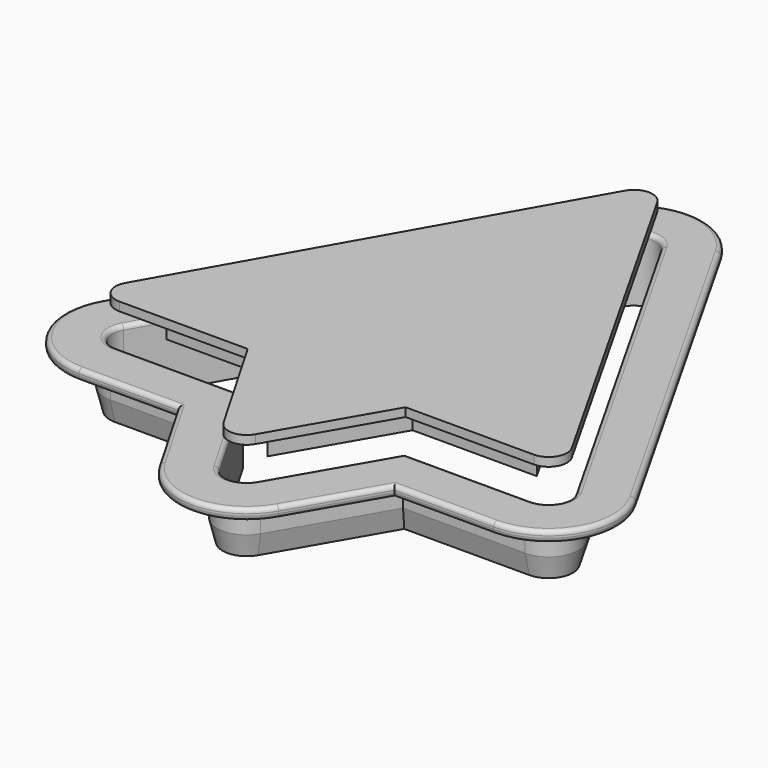
from build123d import *

# Parameters (mm, degrees)
F1_DEPTH     = 2.5
F2_DEPTH     = 15
F0_R         = 2.1252371371
F3_DEPTH     = 15
F4_DEPTH     = 7
F5_T1_DEPTH  = 97.369641179
F5_T3_DEPTH  = 97.369641179
F5_T6_ANGLE  = 119.5382480003
F5_T10_DEPTH = 41.2120527161
F5_T15_DEPTH = 40.6442974674
F5_T18_ANGLE = 120.9235039995
F5_T20_ANGLE = 119.5382480003
F5_T24_DEPTH = 41.2120527161
F5_T29_DEPTH = 40.6442974674
F5_T32_ANGLE = 119.912621019
F5_T37_DEPTH = 40.6442974674
F5_T42_DEPTH = 41.2120527161
F5_T50_DEPTH = 41.2120527161
F5_T55_DEPTH = 40.6442974674
F6_R         = 1
F8_DEPTH     = 25
F9_DEPTH     = 6


# Not quite as in the source:
# - a fillet or chamfer that OpenCascade refuses, or shapes differently, is made with other operations: its cross-section is extruded or revolved along the edge and cut away or added


with BuildPart() as f1:
    # F0 (on Top) → F1 (new body)
    with BuildSketch(Plane.XY):
        with BuildLine():
            Line((65.2872159777, -47.6204884105), (17.2835486697, 37.0937072612))
            ThreePointArc((17.2835486697, 37.0937072612), (3.4454325214, 45.1576695615), (-10.3926836269, 37.0937072612))
            Line((-10.3926836269, 37.0937072612), (-58.3963509349, -47.6204884105))
            ThreePointArc((-58.3963509349, -47.6204884105), (-58.3005499368, -63.4700527455), (-44.5582347866, -71.3673080758))
            Line((-44.5582347866, -71.3673080758), (-21.5553492686, -71.3673080758))
            Line((-21.5553492686, -71.3673080758), (-10.3229719901, -90.7881414994))
            ThreePointArc((-10.3229719901, -90.7881414994), (3.4454325214, -98.7303359177), (17.2138370329, -90.7881414994))
            Line((17.2138370329, -90.7881414994), (28.4462143115, -71.3673080758))
            Line((28.4462143115, -71.3673080758), (51.4490998294, -71.3673080758))
            ThreePointArc((51.4490998294, -71.3673080758), (65.1914149796, -63.4700527455), (65.2872159777, -47.6204884105))
        make_face()
        with BuildLine():
            ThreePointArc((-2.5142515817, 32.629359488), (3.4454325214, 36.1022793142), (9.4051166245, 32.629359488))
            Line((9.4051166245, 32.629359488), (57.4087839325, -52.0848361837))
            ThreePointArc((57.4087839325, -52.0848361837), (57.36752516, -58.9107939655), (51.4490998294, -62.3119178285))
            Line((51.4490998294, -62.3119178285), (23.2226846121, -62.3119178285))
            Line((23.2226846121, -62.3119178285), (9.3750937999, -86.254467817))
            ThreePointArc((9.3750937999, -86.254467817), (3.4454325214, -89.6749456705), (-2.4842287571, -86.254467817))
            Line((-2.4842287571, -86.254467817), (-16.3318195693, -62.3119178285))
            Line((-16.3318195693, -62.3119178285), (-44.5582347866, -62.3119178285))
            ThreePointArc((-44.5582347866, -62.3119178285), (-50.4766601172, -58.9107939655), (-50.5179188897, -52.0848361837))
            Line((-50.5179188897, -52.0848361837), (-2.5142515817, 32.629359488))
        make_face(mode=Mode.SUBTRACT)
    extrude(amount=-F1_DEPTH)

    # F0 (on Top) → F2 (join)
    with BuildSketch(Plane.XY):
        with BuildLine():
            Line((57.4087839325, -52.0848361837), (9.4051166245, 32.629359488))
            ThreePointArc((9.4051166245, 32.629359488), (3.4454325214, 36.1022793142), (-2.5142515817, 32.629359488))
            Line((-2.5142515817, 32.629359488), (-50.5179188897, -52.0848361837))
            ThreePointArc((-50.5179188897, -52.0848361837), (-50.4766601172, -58.9107939655), (-44.5582347866, -62.3119178285))
            Line((-44.5582347866, -62.3119178285), (-16.3318195693, -62.3119178285))
            Line((-16.3318195693, -62.3119178285), (-2.4842287571, -86.254467817))
            ThreePointArc((-2.4842287571, -86.254467817), (3.4454325214, -89.6749456705), (9.3750937999, -86.254467817))
            Line((9.3750937999, -86.254467817), (23.2226846121, -62.3119178285))
            Line((23.2226846121, -62.3119178285), (51.4490998294, -62.3119178285))
            ThreePointArc((51.4490998294, -62.3119178285), (57.36752516, -58.9107939655), (57.4087839325, -52.0848361837))
        make_face()
        with BuildLine():
            ThreePointArc((-0.9047013933, 31.7173008756), (3.4454325214, 34.2522785787), (7.7955664361, 31.7173008756))
            Line((7.7955664361, 31.7173008756), (55.7992337441, -52.9968947961))
            ThreePointArc((55.7992337441, -52.9968947961), (55.769117855, -57.9793451968), (51.4490998294, -60.461917093))
            Line((51.4490998294, -60.461917093), (22.155526431, -60.461917093))
            Line((22.155526431, -60.461917093), (7.773651968, -85.3282460399))
            ThreePointArc((7.773651968, -85.3282460399), (3.4454325214, -87.8249449349), (-0.8827869252, -85.3282460399))
            Line((-0.8827869252, -85.3282460399), (-15.2646613882, -60.461917093))
            Line((-15.2646613882, -60.461917093), (-44.5582347866, -60.461917093))
            ThreePointArc((-44.5582347866, -60.461917093), (-48.8782528122, -57.9793451968), (-48.9083687013, -52.9968947961))
            Line((-48.9083687013, -52.9968947961), (-0.9047013933, 31.7173008756))
        make_face(mode=Mode.SUBTRACT)
    extrude(amount=-F2_DEPTH)

    # F5: chamfer of 5 x 1.25 on 10 edges, made by hand

    # F5_s2 → F5_t1 (cut)
    with BuildSketch(Plane(origin=(13.3845186224, 23.6202522252, 0), x_dir=(0, 0, 1), z_dir=(-0.4930044594, -0.8700267829, 0))):
        Polygon((-10, 18.273885949), (-15, 17.023885949), (-15, 18.273885949), align=None)
    extrude(amount=F5_T1_DEPTH, mode=Mode.SUBTRACT)

    # F5_s4 → F5_t3 (cut)
    with BuildSketch(Plane(origin=(36.2939968422, -64.0496220939, 0), x_dir=(0, 0, 1), z_dir=(-0.4930044594, 0.8700267829, 0))):
        Polygon((-10, 24.2691230939), (-15, 23.0191230939), (-15, 24.2691230939), align=None)
    extrude(amount=F5_T3_DEPTH, mode=Mode.SUBTRACT)

    # F5_s5 → F5_t6 (revolve, cut)
    with BuildSketch(Plane(origin=(-34.6191486856, -61.0939434465, 0), x_dir=(0, 0, 1), z_dir=(0.4930044594, 0.8700267829, 0))):
        Polygon((-10, -18.273885949), (-15, -17.023885949), (-15, -18.273885949), align=None)
    revolve(axis=Axis((-44.5582347866, -55.461917093, -15), (0, 0, 1)), revolution_arc=F5_T6_ANGLE, mode=Mode.SUBTRACT)


with BuildPart() as f3:
    # F0 (on Top) → F3 (new body)
    with BuildSketch(Plane.XY):
        with BuildLine():
            Line((55.7992337441, -52.9968947961), (7.7955664361, 31.7173008756))
            ThreePointArc((7.7955664361, 31.7173008756), (3.4454325214, 34.2522785787), (-0.9047013933, 31.7173008756))
            Line((-0.9047013933, 31.7173008756), (-48.9083687013, -52.9968947961))
            ThreePointArc((-48.9083687013, -52.9968947961), (-48.8782528122, -57.9793451968), (-44.5582347866, -60.461917093))
            Line((-44.5582347866, -60.461917093), (-15.2646613882, -60.461917093))
            Line((-15.2646613882, -60.461917093), (-0.8827869252, -85.3282460399))
            ThreePointArc((-0.8827869252, -85.3282460399), (3.4454325214, -87.8249449349), (7.773651968, -85.3282460399))
            Line((7.773651968, -85.3282460399), (22.155526431, -60.461917093))
            Line((22.155526431, -60.461917093), (51.4490998294, -60.461917093))
            ThreePointArc((51.4490998294, -60.461917093), (55.769117855, -57.9793451968), (55.7992337441, -52.9968947961))
        make_face()
        Polygon((-39.4101028585, -52.4619175743), (3.4454325214, 23.1671418995), (46.3009679013, -52.4619175743), (17.5407904627, -52.4619175743), (3.4454325214, -76.8328581005), (-10.6499254199, -52.4619175743), align=None, mode=Mode.SUBTRACT)
        Polygon((46.3009679013, -52.4619175743), (3.4454325214, 23.1671418995), (-39.4101028585, -52.4619175743), (-10.6499254199, -52.4619175743), (3.4454325214, -76.8328581005), (17.5407904627, -52.4619175743), align=None)
        Polygon((-35.3587796887, -50.1010675165), (3.4454325214, 18.3784427043), (42.2496447315, -50.1010675165), (16.1789529211, -50.1010675165), (3.4454325214, -72.1173844943), (-9.2880878783, -50.1010675165), align=None, mode=Mode.SUBTRACT)
        Polygon((42.2496447315, -50.1010675165), (3.4454325214, 18.3784427043), (-35.3587796887, -50.1010675165), (-9.2880878783, -50.1010675165), (3.4454325214, -72.1173844943), (16.1789529211, -50.1010675165), align=None)
        with Locations((-14.878096059, -27.4075604975)):
            Circle(F0_R, mode=Mode.SUBTRACT)
        Polygon((-12.8765748814, -42.689666152), (-12.8765748814, -35.4246795177), (-11.767576843, -35.4246795177), (-9.1813210194, -41.2681277739), (-6.5903947689, -35.4246795177), (-5.4648038931, -35.4246795177), (-5.4648038931, -42.689666152), (-6.3942293637, -42.689666152), (-6.3942293637, -36.9316674769), (-8.9472681284, -42.689666152), (-9.4033638015, -42.689666152), (-11.9518004358, -36.9316674769), (-11.9518004358, -42.689666152), align=None, mode=Mode.SUBTRACT)
        Polygon((-2.7839182876, -42.689666152), (-3.7133437581, -42.689666152), (-3.7133437581, -35.4246795177), (-2.5877528824, -35.4246795177), (0.0031733681, -41.2681277739), (2.5894291918, -35.4246795177), (3.6984272301, -35.4246795177), (3.6984272301, -42.689666152), (2.7736527845, -42.689666152), (2.7736527845, -36.9316674769), (0.2252161503, -42.689666152), (-0.2308795229, -42.689666152), (-2.7839182876, -36.9316674769), align=None, mode=Mode.SUBTRACT)
        Polygon((7.0893075317, -39.0533059835), (4.8316721804, -35.4246795177), (5.9392736293, -35.4246795177), (7.673623506, -38.402441889), (9.4814058393, -35.4246795177), (10.5444919318, -35.4246795177), (8.2598868757, -39.0533059835), (10.5607574806, -42.689666152), (9.4446605071, -42.689666152), (7.6309749857, -39.6361723542), (5.8071413077, -42.689666152), (4.6372665092, -42.689666152), align=None, mode=Mode.SUBTRACT)
        Polygon((10.8218248934, -36.2534187734), (10.8218248934, -35.4246795177), (13.1533117965, -35.4246795177), (13.1533117965, -36.2534187734), (12.4322017655, -36.2534187734), (12.4322017655, -41.8955646455), (13.1625505164, -41.8955646455), (13.1625505164, -42.689666152), (10.8218248934, -42.689666152), (10.8218248934, -41.8955646455), (11.5015460178, -41.8955646455), (11.5015460178, -36.2534187734), align=None, mode=Mode.SUBTRACT)
        Polygon((16.0190779716, -42.689666152), (13.3707774803, -35.4246795177), (14.4054275006, -35.4246795177), (16.5070295334, -41.5401048958), (18.6662711203, -35.4246795177), (19.673185423, -35.4246795177), (16.9846378267, -42.689666152), align=None, mode=Mode.SUBTRACT)
        with Locations((21.7689611018, -27.4075604975)):
            Circle(F0_R, mode=Mode.SUBTRACT)
        with BuildLine():
            Line((-7.565066684, -27.4075604975), (-7.565066684, -11.1319441348))
            Line((-7.565066684, -11.1319441348), (-2.4298110511, -11.1319441348))
            add(Edge.make_bspline(
                [(-2.4298110511, -11.1319441348), (-2.3662628859, -11.1277319227), (-2.1761521622, -11.1151306665), (-1.2327957206, -11.2783416604), (-0.5211634317, -11.547496959), (0.2299466047, -11.9524717121), (0.7848702041, -12.4353144963), (1.2318193278, -13.0031014274), (1.5460073362, -13.6587083311), (1.6843174255, -14.3229828977), (1.7077365425, -15.0653349157), (1.646054142, -15.8432341211), (1.1886971111, -17.0127703282), (0.6250596434, -17.7036813267), (-0.2627651619, -18.4198849126), (-0.854730177, -18.6291207008), (-1.1375576723, -18.729088828)],
                knots=[0, 0, 0, 0, 0.0388828811, 0.1163220472, 0.1889199067, 0.2620977169, 0.3309604833, 0.3989173697, 0.4669571129, 0.5329803689, 0.6011841527, 0.6727074701, 0.7614150711, 0.8383080917, 0.9227472633, 1, 1, 1, 1], degree=3))
            add(Edge.make_bspline(
                [(-1.1375576723, -18.729088828), (-0.9671856539, -18.7514978709), (-0.6033813766, -18.7993490718), (0.0660586896, -18.9816127322), (0.6010266046, -19.2327583636), (1.0741312431, -19.5553602716), (1.5414018503, -19.9423331016), (1.9346472569, -20.4967262682), (2.2833861826, -21.1276117238), (2.4839790815, -21.8883826229), (2.5094475477, -22.8489771807), (2.4496384326, -23.6991497175), (2.1576362149, -24.5725173863), (1.7392478578, -25.3275471294), (1.0558605738, -26.0802068889), (0.2202330448, -26.6918164691), (-0.9200115081, -27.1863840995), (-2.0235119167, -27.3699531875), (-2.5665856599, -27.3958136895), (-2.8132700827, -27.4075604975)],
                knots=[0, 0, 0, 0, 0.0479736496, 0.1024406419, 0.1529437174, 0.2021509478, 0.2529493227, 0.306782996, 0.3621148536, 0.4200783659, 0.4840983738, 0.544859907, 0.6069989637, 0.6678698662, 0.7332197146, 0.7999838456, 0.8730818232, 0.9423490132, 1, 1, 1, 1], degree=3))
            Line((-2.8132700827, -27.4075604975), (-7.565066684, -27.4075604975))
        make_face(mode=Mode.SUBTRACT)
        Polygon((7.5685675256, -27.4075604975), (7.5685675256, -11.1319441348), (15.8298257738, -11.1319441348), (15.8298257738, -12.9275834188), (9.5347687602, -12.9275834188), (9.5347687602, -18.4326544404), (15.3840826824, -18.4326544404), (15.3840826824, -20.2224254608), (9.5347687602, -20.2224254608), (9.5347687602, -27.4075604975), align=None, mode=Mode.SUBTRACT)
        with BuildLine():
            Line((-2.4298110511, -11.1319441348), (-7.565066684, -11.1319441348))
            Line((-7.565066684, -11.1319441348), (-7.565066684, -27.4075604975))
            Line((-7.565066684, -27.4075604975), (-2.8132700827, -27.4075604975))
            add(Edge.make_bspline(
                [(-1.1375576723, -18.729088828), (-0.9671856539, -18.7514978709), (-0.6033813766, -18.7993490718), (0.0660586896, -18.9816127322), (0.6010266046, -19.2327583636), (1.0741312431, -19.5553602716), (1.5414018503, -19.9423331016), (1.9346472569, -20.4967262682), (2.2833861826, -21.1276117238), (2.4839790815, -21.8883826229), (2.5094475477, -22.8489771807), (2.4496384326, -23.6991497175), (2.1576362149, -24.5725173863), (1.7392478578, -25.3275471294), (1.0558605738, -26.0802068889), (0.2202330448, -26.6918164691), (-0.9200115081, -27.1863840995), (-2.0235119167, -27.3699531875), (-2.5665856599, -27.3958136895), (-2.8132700827, -27.4075604975)],
                knots=[0, 0, 0, 0, 0.0479736496, 0.1024406419, 0.1529437174, 0.2021509478, 0.2529493227, 0.306782996, 0.3621148536, 0.4200783659, 0.4840983738, 0.544859907, 0.6069989637, 0.6678698662, 0.7332197146, 0.7999838456, 0.8730818232, 0.9423490132, 1, 1, 1, 1], degree=3))
            add(Edge.make_bspline(
                [(-2.4298110511, -11.1319441348), (-2.3662628859, -11.1277319227), (-2.1761521622, -11.1151306665), (-1.2327957206, -11.2783416604), (-0.5211634317, -11.547496959), (0.2299466047, -11.9524717121), (0.7848702041, -12.4353144963), (1.2318193278, -13.0031014274), (1.5460073362, -13.6587083311), (1.6843174255, -14.3229828977), (1.7077365425, -15.0653349157), (1.646054142, -15.8432341211), (1.1886971111, -17.0127703282), (0.6250596434, -17.7036813267), (-0.2627651619, -18.4198849126), (-0.854730177, -18.6291207008), (-1.1375576723, -18.729088828)],
                knots=[0, 0, 0, 0, 0.0388828811, 0.1163220472, 0.1889199067, 0.2620977169, 0.3309604833, 0.3989173697, 0.4669571129, 0.5329803689, 0.6011841527, 0.6727074701, 0.7614150711, 0.8383080917, 0.9227472633, 1, 1, 1, 1], degree=3))
        make_face()
        with BuildLine():
            Line((-5.58487745, -19.8434796184), (-3.307457082, -19.8434796184))
            add(Edge.make_bspline(
                [(-3.307457082, -19.8434796184), (-3.2498357835, -19.8428036642), (-3.0860007795, -19.8408817192), (-2.3799055918, -19.8654680454), (-1.6268851064, -20.0042335871), (-1.019466756, -20.2480680307), (-0.5697062953, -20.5128451486), (-0.07437245, -20.9142139222), (0.2953084647, -21.5455618329), (0.4441260994, -22.1066423066), (0.4757687104, -22.8954768575), (0.3980948825, -23.575306673), (0.075616609, -24.2468728091), (-0.3508103129, -24.7690471447), (-0.9760984475, -25.2180768852), (-1.7961336582, -25.5140032725), (-2.5338206103, -25.6052764347), (-2.7822168208, -25.5967711127), (-2.8820293956, -25.5933534354)],
                knots=[0, 0, 0, 0, 0.0354857234, 0.1008967829, 0.1714114002, 0.2342692197, 0.2906085395, 0.3530234902, 0.4194127533, 0.4794737535, 0.5485734468, 0.6139414763, 0.6807808741, 0.7449692549, 0.8132796881, 0.8874962971, 0.954792852, 1, 1, 1, 1], degree=3))
            Line((-2.8820293956, -25.5933534354), (-5.58487745, -25.5933534354))
            Line((-5.58487745, -25.5933534354), (-5.58487745, -19.8434796184))
        make_face(mode=Mode.SUBTRACT)
        with BuildLine():
            Line((-5.58487745, -12.8929018974), (-2.9470350128, -12.8929018974))
            add(Edge.make_bspline(
                [(-2.9470350128, -12.8929018974), (-2.4131396785, -12.8929018974), (-1.5432901024, -13.1842615684), (-0.7077008555, -13.7752698817), (-0.3260399258, -14.700881483), (-0.3463416279, -15.7301453564), (-0.5657422377, -16.5535994965), (-1.0246612964, -17.2014411368), (-1.7455701765, -17.7112813131), (-2.3902032572, -17.9571104394), (-3.2757078506, -18.0818341563), (-3.5074716434, -18.0677678436), (-3.6531293299, -18.0677678436)],
                knots=[0, 0, 0, 0, 0.1294375653, 0.2356659509, 0.3404986069, 0.4492768475, 0.5477671899, 0.6427411456, 0.7421875316, 0.8338204464, 0.9329618949, 1, 1, 1, 1], degree=3))
            Line((-3.6531293299, -18.0677678436), (-5.58487745, -18.0677678436))
            Line((-5.58487745, -18.0677678436), (-5.58487745, -12.8929018974))
        make_face(mode=Mode.SUBTRACT)
        Polygon((15.8298257738, -11.1319441348), (7.5685675256, -11.1319441348), (7.5685675256, -27.4075604975), (9.5347687602, -27.4075604975), (9.5347687602, -20.2224254608), (15.3840826824, -20.2224254608), (15.3840826824, -18.4326544404), (9.5347687602, -18.4326544404), (9.5347687602, -12.9275834188), (15.8298257738, -12.9275834188), align=None)
        with BuildLine():
            add(Edge.make_bspline(
                [(-3.307457082, -19.8434796184), (-3.2498357835, -19.8428036642), (-3.0860007795, -19.8408817192), (-2.3799055918, -19.8654680454), (-1.6268851064, -20.0042335871), (-1.019466756, -20.2480680307), (-0.5697062953, -20.5128451486), (-0.07437245, -20.9142139222), (0.2953084647, -21.5455618329), (0.4441260994, -22.1066423066), (0.4757687104, -22.8954768575), (0.3980948825, -23.575306673), (0.075616609, -24.2468728091), (-0.3508103129, -24.7690471447), (-0.9760984475, -25.2180768852), (-1.7961336582, -25.5140032725), (-2.5338206103, -25.6052764347), (-2.7822168208, -25.5967711127), (-2.8820293956, -25.5933534354)],
                knots=[0, 0, 0, 0, 0.0354857234, 0.1008967829, 0.1714114002, 0.2342692197, 0.2906085395, 0.3530234902, 0.4194127533, 0.4794737535, 0.5485734468, 0.6139414763, 0.6807808741, 0.7449692549, 0.8132796881, 0.8874962971, 0.954792852, 1, 1, 1, 1], degree=3))
            Line((-3.307457082, -19.8434796184), (-5.58487745, -19.8434796184))
            Line((-5.58487745, -19.8434796184), (-5.58487745, -25.5933534354))
            Line((-5.58487745, -25.5933534354), (-2.8820293956, -25.5933534354))
        make_face()
        with BuildLine():
            add(Edge.make_bspline(
                [(-2.9470350128, -12.8929018974), (-2.4131396785, -12.8929018974), (-1.5432901024, -13.1842615684), (-0.7077008555, -13.7752698817), (-0.3260399258, -14.700881483), (-0.3463416279, -15.7301453564), (-0.5657422377, -16.5535994965), (-1.0246612964, -17.2014411368), (-1.7455701765, -17.7112813131), (-2.3902032572, -17.9571104394), (-3.2757078506, -18.0818341563), (-3.5074716434, -18.0677678436), (-3.6531293299, -18.0677678436)],
                knots=[0, 0, 0, 0, 0.1294375653, 0.2356659509, 0.3404986069, 0.4492768475, 0.5477671899, 0.6427411456, 0.7421875316, 0.8338204464, 0.9329618949, 1, 1, 1, 1], degree=3))
            Line((-2.9470350128, -12.8929018974), (-5.58487745, -12.8929018974))
            Line((-5.58487745, -12.8929018974), (-5.58487745, -18.0677678436))
            Line((-5.58487745, -18.0677678436), (-3.6531293299, -18.0677678436))
        make_face()
        Polygon((-11.767576843, -35.4246795177), (-12.8765748814, -35.4246795177), (-12.8765748814, -42.689666152), (-11.9518004358, -42.689666152), (-11.9518004358, -36.9316674769), (-9.4033638015, -42.689666152), (-8.9472681284, -42.689666152), (-6.3942293637, -36.9316674769), (-6.3942293637, -42.689666152), (-5.4648038931, -42.689666152), (-5.4648038931, -35.4246795177), (-6.5903947689, -35.4246795177), (-9.1813210194, -41.2681277739), align=None)
        Polygon((-3.7133437581, -35.4246795177), (-3.7133437581, -42.689666152), (-2.7839182876, -42.689666152), (-2.7839182876, -36.9316674769), (-0.2308795229, -42.689666152), (0.2252161503, -42.689666152), (2.7736527845, -36.9316674769), (2.7736527845, -42.689666152), (3.6984272301, -42.689666152), (3.6984272301, -35.4246795177), (2.5894291918, -35.4246795177), (0.0031733681, -41.2681277739), (-2.5877528824, -35.4246795177), align=None)
        Polygon((5.9392736293, -35.4246795177), (4.8316721804, -35.4246795177), (7.0893075317, -39.0533059835), (4.6372665092, -42.689666152), (5.8071413077, -42.689666152), (7.6309749857, -39.6361723542), (9.4446605071, -42.689666152), (10.5607574806, -42.689666152), (8.2598868757, -39.0533059835), (10.5444919318, -35.4246795177), (9.4814058393, -35.4246795177), (7.673623506, -38.402441889), align=None)
        with Locations((-14.878096059, -27.4075604975)):
            Circle(F0_R)
        with Locations((21.7689611018, -27.4075604975)):
            Circle(F0_R)
        Polygon((14.4054275006, -35.4246795177), (13.3707774803, -35.4246795177), (16.0190779716, -42.689666152), (16.9846378267, -42.689666152), (19.673185423, -35.4246795177), (18.6662711203, -35.4246795177), (16.5070295334, -41.5401048958), align=None)
        Polygon((13.1533117965, -35.4246795177), (10.8218248934, -35.4246795177), (10.8218248934, -36.2534187734), (11.5015460178, -36.2534187734), (11.5015460178, -41.8955646455), (10.8218248934, -41.8955646455), (10.8218248934, -42.689666152), (13.1625505164, -42.689666152), (13.1625505164, -41.8955646455), (12.4322017655, -41.8955646455), (12.4322017655, -36.2534187734), (13.1533117965, -36.2534187734), align=None)
    extrude(amount=F3_DEPTH)

    # F0 (on Top) → F4 (cut)
    with BuildSketch(Plane.XY):
        with BuildLine():
            Line((55.7992337441, -52.9968947961), (7.7955664361, 31.7173008756))
            ThreePointArc((7.7955664361, 31.7173008756), (3.4454325214, 34.2522785787), (-0.9047013933, 31.7173008756))
            Line((-0.9047013933, 31.7173008756), (-48.9083687013, -52.9968947961))
            ThreePointArc((-48.9083687013, -52.9968947961), (-48.8782528122, -57.9793451968), (-44.5582347866, -60.461917093))
            Line((-44.5582347866, -60.461917093), (-15.2646613882, -60.461917093))
            Line((-15.2646613882, -60.461917093), (-0.8827869252, -85.3282460399))
            ThreePointArc((-0.8827869252, -85.3282460399), (3.4454325214, -87.8249449349), (7.773651968, -85.3282460399))
            Line((7.773651968, -85.3282460399), (22.155526431, -60.461917093))
            Line((22.155526431, -60.461917093), (51.4490998294, -60.461917093))
            ThreePointArc((51.4490998294, -60.461917093), (55.769117855, -57.9793451968), (55.7992337441, -52.9968947961))
        make_face()
        Polygon((-39.4101028585, -52.4619175743), (3.4454325214, 23.1671418995), (46.3009679013, -52.4619175743), (17.5407904627, -52.4619175743), (3.4454325214, -76.8328581005), (-10.6499254199, -52.4619175743), align=None, mode=Mode.SUBTRACT)
        Polygon((42.2496447315, -50.1010675165), (3.4454325214, 18.3784427043), (-35.3587796887, -50.1010675165), (-9.2880878783, -50.1010675165), (3.4454325214, -72.1173844943), (16.1789529211, -50.1010675165), align=None)
        with Locations((-14.878096059, -27.4075604975)):
            Circle(F0_R, mode=Mode.SUBTRACT)
        Polygon((-12.8765748814, -42.689666152), (-12.8765748814, -35.4246795177), (-11.767576843, -35.4246795177), (-9.1813210194, -41.2681277739), (-6.5903947689, -35.4246795177), (-5.4648038931, -35.4246795177), (-5.4648038931, -42.689666152), (-6.3942293637, -42.689666152), (-6.3942293637, -36.9316674769), (-8.9472681284, -42.689666152), (-9.4033638015, -42.689666152), (-11.9518004358, -36.9316674769), (-11.9518004358, -42.689666152), align=None, mode=Mode.SUBTRACT)
        Polygon((-2.7839182876, -42.689666152), (-3.7133437581, -42.689666152), (-3.7133437581, -35.4246795177), (-2.5877528824, -35.4246795177), (0.0031733681, -41.2681277739), (2.5894291918, -35.4246795177), (3.6984272301, -35.4246795177), (3.6984272301, -42.689666152), (2.7736527845, -42.689666152), (2.7736527845, -36.9316674769), (0.2252161503, -42.689666152), (-0.2308795229, -42.689666152), (-2.7839182876, -36.9316674769), align=None, mode=Mode.SUBTRACT)
        Polygon((7.0893075317, -39.0533059835), (4.8316721804, -35.4246795177), (5.9392736293, -35.4246795177), (7.673623506, -38.402441889), (9.4814058393, -35.4246795177), (10.5444919318, -35.4246795177), (8.2598868757, -39.0533059835), (10.5607574806, -42.689666152), (9.4446605071, -42.689666152), (7.6309749857, -39.6361723542), (5.8071413077, -42.689666152), (4.6372665092, -42.689666152), align=None, mode=Mode.SUBTRACT)
        Polygon((10.8218248934, -36.2534187734), (10.8218248934, -35.4246795177), (13.1533117965, -35.4246795177), (13.1533117965, -36.2534187734), (12.4322017655, -36.2534187734), (12.4322017655, -41.8955646455), (13.1625505164, -41.8955646455), (13.1625505164, -42.689666152), (10.8218248934, -42.689666152), (10.8218248934, -41.8955646455), (11.5015460178, -41.8955646455), (11.5015460178, -36.2534187734), align=None, mode=Mode.SUBTRACT)
        Polygon((16.0190779716, -42.689666152), (13.3707774803, -35.4246795177), (14.4054275006, -35.4246795177), (16.5070295334, -41.5401048958), (18.6662711203, -35.4246795177), (19.673185423, -35.4246795177), (16.9846378267, -42.689666152), align=None, mode=Mode.SUBTRACT)
        with Locations((21.7689611018, -27.4075604975)):
            Circle(F0_R, mode=Mode.SUBTRACT)
        with BuildLine():
            Line((-7.565066684, -27.4075604975), (-7.565066684, -11.1319441348))
            Line((-7.565066684, -11.1319441348), (-2.4298110511, -11.1319441348))
            add(Edge.make_bspline(
                [(-2.4298110511, -11.1319441348), (-2.3662628859, -11.1277319227), (-2.1761521622, -11.1151306665), (-1.2327957206, -11.2783416604), (-0.5211634317, -11.547496959), (0.2299466047, -11.9524717121), (0.7848702041, -12.4353144963), (1.2318193278, -13.0031014274), (1.5460073362, -13.6587083311), (1.6843174255, -14.3229828977), (1.7077365425, -15.0653349157), (1.646054142, -15.8432341211), (1.1886971111, -17.0127703282), (0.6250596434, -17.7036813267), (-0.2627651619, -18.4198849126), (-0.854730177, -18.6291207008), (-1.1375576723, -18.729088828)],
                knots=[0, 0, 0, 0, 0.0388828811, 0.1163220472, 0.1889199067, 0.2620977169, 0.3309604833, 0.3989173697, 0.4669571129, 0.5329803689, 0.6011841527, 0.6727074701, 0.7614150711, 0.8383080917, 0.9227472633, 1, 1, 1, 1], degree=3))
            add(Edge.make_bspline(
                [(-1.1375576723, -18.729088828), (-0.9671856539, -18.7514978709), (-0.6033813766, -18.7993490718), (0.0660586896, -18.9816127322), (0.6010266046, -19.2327583636), (1.0741312431, -19.5553602716), (1.5414018503, -19.9423331016), (1.9346472569, -20.4967262682), (2.2833861826, -21.1276117238), (2.4839790815, -21.8883826229), (2.5094475477, -22.8489771807), (2.4496384326, -23.6991497175), (2.1576362149, -24.5725173863), (1.7392478578, -25.3275471294), (1.0558605738, -26.0802068889), (0.2202330448, -26.6918164691), (-0.9200115081, -27.1863840995), (-2.0235119167, -27.3699531875), (-2.5665856599, -27.3958136895), (-2.8132700827, -27.4075604975)],
                knots=[0, 0, 0, 0, 0.0479736496, 0.1024406419, 0.1529437174, 0.2021509478, 0.2529493227, 0.306782996, 0.3621148536, 0.4200783659, 0.4840983738, 0.544859907, 0.6069989637, 0.6678698662, 0.7332197146, 0.7999838456, 0.8730818232, 0.9423490132, 1, 1, 1, 1], degree=3))
            Line((-2.8132700827, -27.4075604975), (-7.565066684, -27.4075604975))
        make_face(mode=Mode.SUBTRACT)
        Polygon((7.5685675256, -27.4075604975), (7.5685675256, -11.1319441348), (15.8298257738, -11.1319441348), (15.8298257738, -12.9275834188), (9.5347687602, -12.9275834188), (9.5347687602, -18.4326544404), (15.3840826824, -18.4326544404), (15.3840826824, -20.2224254608), (9.5347687602, -20.2224254608), (9.5347687602, -27.4075604975), align=None, mode=Mode.SUBTRACT)
        with BuildLine():
            add(Edge.make_bspline(
                [(-3.307457082, -19.8434796184), (-3.2498357835, -19.8428036642), (-3.0860007795, -19.8408817192), (-2.3799055918, -19.8654680454), (-1.6268851064, -20.0042335871), (-1.019466756, -20.2480680307), (-0.5697062953, -20.5128451486), (-0.07437245, -20.9142139222), (0.2953084647, -21.5455618329), (0.4441260994, -22.1066423066), (0.4757687104, -22.8954768575), (0.3980948825, -23.575306673), (0.075616609, -24.2468728091), (-0.3508103129, -24.7690471447), (-0.9760984475, -25.2180768852), (-1.7961336582, -25.5140032725), (-2.5338206103, -25.6052764347), (-2.7822168208, -25.5967711127), (-2.8820293956, -25.5933534354)],
                knots=[0, 0, 0, 0, 0.0354857234, 0.1008967829, 0.1714114002, 0.2342692197, 0.2906085395, 0.3530234902, 0.4194127533, 0.4794737535, 0.5485734468, 0.6139414763, 0.6807808741, 0.7449692549, 0.8132796881, 0.8874962971, 0.954792852, 1, 1, 1, 1], degree=3))
            Line((-3.307457082, -19.8434796184), (-5.58487745, -19.8434796184))
            Line((-5.58487745, -19.8434796184), (-5.58487745, -25.5933534354))
            Line((-5.58487745, -25.5933534354), (-2.8820293956, -25.5933534354))
        make_face()
        with BuildLine():
            add(Edge.make_bspline(
                [(-2.9470350128, -12.8929018974), (-2.4131396785, -12.8929018974), (-1.5432901024, -13.1842615684), (-0.7077008555, -13.7752698817), (-0.3260399258, -14.700881483), (-0.3463416279, -15.7301453564), (-0.5657422377, -16.5535994965), (-1.0246612964, -17.2014411368), (-1.7455701765, -17.7112813131), (-2.3902032572, -17.9571104394), (-3.2757078506, -18.0818341563), (-3.5074716434, -18.0677678436), (-3.6531293299, -18.0677678436)],
                knots=[0, 0, 0, 0, 0.1294375653, 0.2356659509, 0.3404986069, 0.4492768475, 0.5477671899, 0.6427411456, 0.7421875316, 0.8338204464, 0.9329618949, 1, 1, 1, 1], degree=3))
            Line((-2.9470350128, -12.8929018974), (-5.58487745, -12.8929018974))
            Line((-5.58487745, -12.8929018974), (-5.58487745, -18.0677678436))
            Line((-5.58487745, -18.0677678436), (-3.6531293299, -18.0677678436))
        make_face()
    extrude(amount=F4_DEPTH, mode=Mode.SUBTRACT)

    # F7 (on face) → F8 (cut)
    with BuildSketch(Plane.XY.offset(15)):
        with BuildLine():
            Line((22.155526431, -60.461917093), (51.4490998294, -60.461917093))
            ThreePointArc((51.4490998294, -60.461917093), (55.769117855, -57.9793451968), (55.7992337441, -52.9968947961))
            Line((55.7992337441, -52.9968947961), (7.7955664361, 31.7173008756))
            ThreePointArc((7.7955664361, 31.7173008756), (3.4454325214, 34.2522785787), (-0.9047013933, 31.7173008756))
            Line((-0.9047013933, 31.7173008756), (-48.9083687013, -52.9968947961))
            ThreePointArc((-48.9083687013, -52.9968947961), (-48.8782528122, -57.9793451968), (-44.5582347866, -60.461917093))
            Line((-44.5582347866, -60.461917093), (-15.2646613882, -60.461917093))
            Line((-15.2646613882, -60.461917093), (-0.8827869252, -85.3282460399))
            ThreePointArc((-0.8827869252, -85.3282460399), (3.4454325214, -87.8249449349), (7.773651968, -85.3282460399))
            Line((7.773651968, -85.3282460399), (22.155526431, -60.461917093))
        make_face()
        with BuildLine():
            ThreePointArc((-0.2521813061, 31.347547531), (3.4454325214, 33.5022785787), (7.1430463489, 31.347547531))
            Line((7.1430463489, 31.347547531), (55.1467136569, -53.3666481407))
            ThreePointArc((55.1467136569, -53.3666481407), (55.1211151512, -57.6017309812), (51.4490998294, -59.711917093))
            Line((51.4490998294, -59.711917093), (21.7228949079, -59.711917093))
            Line((21.7228949079, -59.711917093), (7.124419051, -84.9527508742))
            ThreePointArc((7.124419051, -84.9527508742), (3.4454325214, -87.0749449349), (-0.2335540082, -84.9527508742))
            Line((-0.2335540082, -84.9527508742), (-14.8320298651, -59.711917093))
            Line((-14.8320298651, -59.711917093), (-44.5582347866, -59.711917093))
            ThreePointArc((-44.5582347866, -59.711917093), (-48.2302501084, -57.6017309812), (-48.2558486141, -53.3666481407))
            Line((-48.2558486141, -53.3666481407), (-0.2521813061, 31.347547531))
        make_face(mode=Mode.SUBTRACT)
    extrude(amount=-F8_DEPTH, mode=Mode.SUBTRACT)

    # F9 (cut): a face of the model
    f9_faces = [f3.faces().sort_by_distance(p)[0] for p in [
        (3.4454325214, -31.2618112798, 15),
    ]]
    extrude(f9_faces, amount=-F9_DEPTH, mode=Mode.SUBTRACT)


with BuildPart() as f5_tool8:
    # F5_s9 → F5_t10 (new body)
    with BuildSketch(Plane.YZ.offset(-44.5582347866)):
        Polygon((-62.3119178285, -10), (-61.0619178285, -15), (-62.3119178285, -15), align=None)
    extrude(amount=F5_T10_DEPTH)

    split(bisect_by=Plane(origin=(-39.2436526727, -22.697250061, 0), x_dir=(0, 0, 1), z_dir=(-0.8656438893, -0.500660221, 0)), keep=Keep.TOP)


with BuildPart() as f1_1:
    add(f1.part)

    # F5_t7: cut F5_tool8
    add(f5_tool8.part, mode=Mode.SUBTRACT)


with BuildPart() as f5_tool13:
    # F5_s14 → F5_t15 (new body)
    with BuildSketch(Plane(origin=(16.4104409634, -28.3737300177, 0), x_dir=(0, 0, 1), z_dir=(0.500660221, -0.8656438893, 0))):
        Polygon((-10, 45.3346383621), (-15, 44.0846383621), (-15, 45.3346383621), align=None)
    extrude(amount=F5_T15_DEPTH)

    split(bisect_by=Plane.XZ.offset(62.3119178285), keep=Keep.TOP)


with BuildPart() as f1_2:
    add(f1_1.part)

    # F5_t12: cut F5_tool13
    add(f5_tool13.part, mode=Mode.SUBTRACT)

    # F5_s17 → F5_t18 (revolve, cut)
    with BuildSketch(Plane(origin=(-11.7096704658, 20.6645735778, 0), x_dir=(0, 0, 1), z_dir=(0.4930044594, -0.8700267829, 0))):
        Polygon((-10, -24.2691230939), (-15, -23.0191230939), (-15, -24.2691230939), align=None)
    revolve(axis=Axis((3.4454325214, 29.2522785787, -15), (0, 0, 1)), revolution_arc=F5_T18_ANGLE, mode=Mode.SUBTRACT)

    # F5_s19 → F5_t20 (revolve, cut)
    with BuildSketch(Plane.YZ.offset(51.4490998294)):
        Polygon((-62.3119178285, -10), (-61.0619178285, -15), (-62.3119178285, -15), align=None)
    revolve(axis=Axis((51.4490998294, -55.461917093, -15), (0, 0, 1)), revolution_arc=F5_T20_ANGLE, mode=Mode.SUBTRACT)


with BuildPart() as f5_tool22:
    # F5_s23 → F5_t24 (new body)
    with BuildSketch(Plane.YZ.offset(10.2370471133)):
        Polygon((-62.3119178285, -10), (-61.0619178285, -15), (-62.3119178285, -15), align=None)
    extrude(amount=F5_T24_DEPTH)

    split(bisect_by=Plane(origin=(44.4072489573, -25.6837059107, 0), x_dir=(0, 0, 1), z_dir=(0.8656438893, -0.500660221, 0)), keep=Keep.TOP)


with BuildPart() as f1_3:
    add(f1_2.part)

    # F5_t21: cut F5_tool22
    add(f5_tool22.part, mode=Mode.SUBTRACT)


with BuildPart() as f5_tool27:
    # F5_s28 → F5_t29 (new body)
    with BuildSketch(Plane(origin=(-35.0321551574, -60.5707619063, 0), x_dir=(0, 0, 1), z_dir=(0.500660221, 0.8656438893, 0))):
        Polygon((-10, 51.2996735785), (-15, 50.0496735785), (-15, 51.2996735785), align=None)
    extrude(amount=F5_T29_DEPTH)

    split(bisect_by=Plane.XZ.offset(62.3119178285), keep=Keep.TOP)


with BuildPart() as f1_4:
    add(f1_3.part)

    # F5_t26: cut F5_tool27
    add(f5_tool27.part, mode=Mode.SUBTRACT)

    # F5_s31 → F5_t32 (revolve, cut)
    with BuildSketch(Plane(origin=(36.7594239155, -63.557217756, 0), x_dir=(0, 0, 1), z_dir=(-0.500660221, 0.8656438893, 0))):
        Polygon((-10, -45.3346383621), (-15, -44.0846383621), (-15, -45.3346383621), align=None)
    revolve(axis=Axis((3.4454325214, -82.8249449349, -15), (0, 0, 1)), revolution_arc=F5_T32_ANGLE, mode=Mode.SUBTRACT)


with BuildPart() as f5_tool35:
    # F5_s36 → F5_t37 (new body)
    with BuildSketch(Plane(origin=(16.4104409634, -28.3737300177, 0), x_dir=(0, 0, 1), z_dir=(0.500660221, -0.8656438893, 0))):
        Polygon((-10, 45.3346383621), (-15, 44.0846383621), (-15, 45.3346383621), align=None)
    extrude(amount=F5_T37_DEPTH)

    split(bisect_by=Plane.XZ.offset(62.3119178285), keep=Keep.BOTTOM)

    split(bisect_by=Plane.XZ.offset(60.461917093), keep=Keep.TOP)


with BuildPart() as f5_tool40:
    # F5_s41 → F5_t42 (new body)
    with BuildSketch(Plane.YZ.offset(-44.5582347866)):
        Polygon((-62.3119178285, -10), (-61.0619178285, -15), (-62.3119178285, -15), align=None)
    extrude(amount=F5_T42_DEPTH)

    split(bisect_by=Plane(origin=(-39.2436526727, -22.697250061, 0), x_dir=(0, 0, 1), z_dir=(0.8656438893, 0.500660221, 0)), keep=Keep.TOP)

    split(bisect_by=Plane(origin=(-37.6422108407, -21.7710282839, 0), x_dir=(0, 0, 1), z_dir=(-0.8656438893, -0.500660221, 0)), keep=Keep.TOP)


with BuildPart() as f5_tool35_1:
    add(f5_tool35.part)

    # F5_t45: intersect F5_tool40
    add(f5_tool40.part, mode=Mode.INTERSECT)


with BuildPart() as f1_5:
    add(f1_4.part)

    # F5_t33: cut F5_tool35
    add(f5_tool35_1.part, mode=Mode.SUBTRACT)


with BuildPart() as f5_tool48:
    # F5_s49 → F5_t50 (new body)
    with BuildSketch(Plane.YZ.offset(10.2370471133)):
        Polygon((-62.3119178285, -10), (-61.0619178285, -15), (-62.3119178285, -15), align=None)
    extrude(amount=F5_T50_DEPTH)

    split(bisect_by=Plane(origin=(44.4072489573, -25.6837059107, 0), x_dir=(0, 0, 1), z_dir=(-0.8656438893, 0.500660221, 0)), keep=Keep.TOP)

    split(bisect_by=Plane(origin=(42.8058071254, -24.7574841336, 0), x_dir=(0, 0, 1), z_dir=(0.8656438893, -0.500660221, 0)), keep=Keep.TOP)


with BuildPart() as f5_tool53:
    # F5_s54 → F5_t55 (new body)
    with BuildSketch(Plane(origin=(-35.0321551574, -60.5707619063, 0), x_dir=(0, 0, 1), z_dir=(0.500660221, 0.8656438893, 0))):
        Polygon((-10, 51.2996735785), (-15, 50.0496735785), (-15, 51.2996735785), align=None)
    extrude(amount=F5_T55_DEPTH)

    split(bisect_by=Plane.XZ.offset(62.3119178285), keep=Keep.BOTTOM)

    split(bisect_by=Plane.XZ.offset(60.461917093), keep=Keep.TOP)


with BuildPart() as f5_tool48_1:
    add(f5_tool48.part)

    # F5_t58: intersect F5_tool53
    add(f5_tool53.part, mode=Mode.INTERSECT)


with BuildPart() as f1_6:
    add(f1_5.part)

    # F5_t46: cut F5_tool48
    add(f5_tool48_1.part, mode=Mode.SUBTRACT)

    # F6
    f6_edges = [f1_6.edges().sort_by_distance(p)[0] for p in [
        (-26.516085, -9.727738, -2.5),
        (-34.394517, -5.263391, -2.5),
        (-34.394517, -5.263391, 0),
        (-15.939161, -81.077725, -2.5),
        (-15.939161, -81.077725, 0),
        (31.7974, -10.639797, 0),
        (-8.073724, -72.895082, 0),
        (16.298889, -74.283193, -2.5),
        (65.191415, -63.470053, 0),
        (65.191415, -63.470053, -2.5),
        (41.285382, -5.263391, -2.5),
        (3.445433, 45.15767, -2.5),
        (-58.30055, -63.470053, -2.5),
        (-33.056792, -71.367308, -2.5),
        (3.445433, -98.730336, -2.5),
        (22.830026, -81.077725, -2.5),
        (39.947657, -71.367308, -2.5),
        (3.445433, 36.102279, -2.5),
        (33.40695, -9.727738, -2.5),
        (57.367525, -58.910794, -2.5),
        (37.335892, -62.311918, -2.5),
        (3.445433, -89.674946, -2.5),
        (-9.408024, -74.283193, -2.5),
        (-30.445027, -62.311918, -2.5),
        (-50.47666, -58.910794, -2.5),
        (-24.906535, -10.639797, 0),
        (-48.878253, -57.979345, 0),
        (-29.911448, -60.461917, 0),
        (3.445433, -87.824945, 0),
        (14.964589, -72.895082, 0),
        (36.802313, -60.461917, 0),
        (55.769118, -57.979345, 0),
        (3.445433, 34.252279, 0),
        (22.830026, -81.077725, 0),
        (3.445433, -98.730336, 0),
        (-33.056792, -71.367308, 0),
        (-58.30055, -63.470053, 0),
        (3.445433, 45.15767, 0),
        (41.285382, -5.263391, 0),
        (39.947657, -71.367308, 0),
    ]]
    fillet(f6_edges, radius=F6_R)


solid = Compound([f3.part, f1_6.part])
